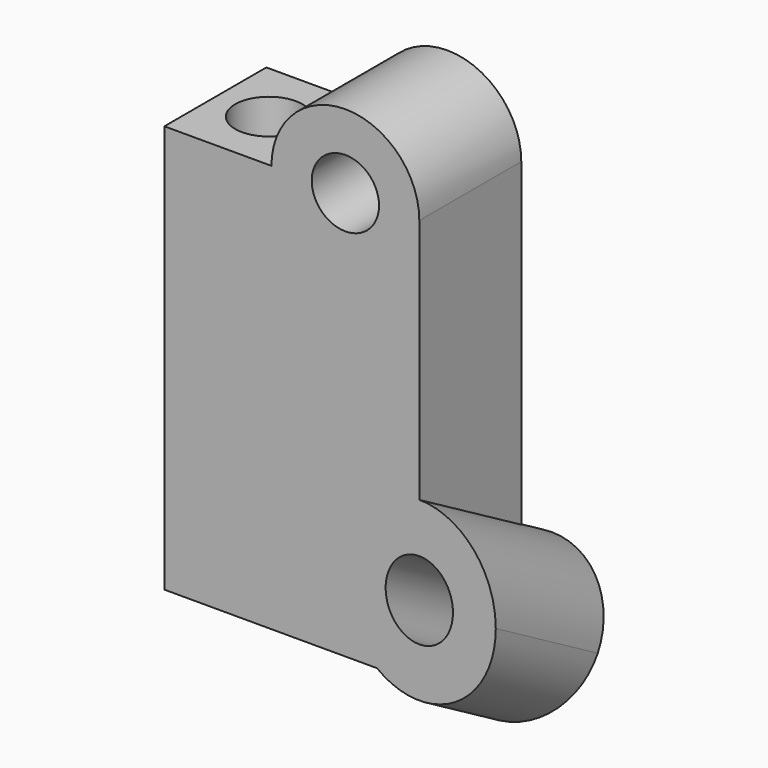
from build123d import *

# Parameters (mm, degrees)
F1_DEPTH        = 25
F3_R            = 15
F4_DEPTH        = 52
F6_D            = 13.2
F6_CBORE_D      = 19.25
F6_CBORE_DEPTH  = 0
F8_D            = 13.2
F8_CBORE_D      = 19.25
F8_CBORE_DEPTH  = 0
F10_D           = 13.2
F10_CBORE_D     = 19.25
F10_CBORE_DEPTH = 0
F11_W           = 35.8968544751
F11_H           = 52.9583077878
F12_DEPTH       = 58


with BuildPart() as f1:
    # F0 (on Front) → F1 (new body)
    with BuildSketch(Plane.XZ):
        with BuildLine():
            Line((-25, -40), (25, -40))
            Line((25, -40), (25, 40))
            ThreePointArc((25, 40), (10.5, 25.5), (-4, 40))
            Line((-4, 40), (-25, 40))
            Line((-25, 40), (-25, -40))
        make_face()
        with BuildLine():
            ThreePointArc((-4, 40), (10.5, 25.5), (25, 40))
            Line((25, 40), (-4, 40))
        make_face()
        with BuildLine():
            Line((-4, 40), (25, 40))
            ThreePointArc((25, 40), (10.5, 54.5), (-4, 40))
        make_face()
    extrude(amount=F1_DEPTH)

    # F3 (on face) → F4 (join)
    with BuildSketch(Plane(origin=(0, 17.3205080757, -10), x_dir=(1, 0, 0), z_dir=(0, -0.8660254038, 0.5))):
        with Locations((25, -34.6410161514)):
            Circle(F3_R)
    extrude(amount=F4_DEPTH)

    # F6 (through all)
    with Locations(Plane(origin=(0, 17.3205080757, -10), x_dir=(-1, 0, 0), z_dir=(0, 0.8660254038, -0.5))):
        with Locations((-25, -34.6410161514)):
            CounterBoreHole(F6_D / 2, F6_CBORE_D / 2, F6_CBORE_DEPTH)

    # F8 (through all)
    with Locations(Plane(origin=(0, 0, 0), x_dir=(-1, 0, 0), z_dir=(0, 1, 0))):
        with Locations((-10.5, 40)):
            CounterBoreHole(F8_D / 2, F8_CBORE_D / 2, F8_CBORE_DEPTH)

    # F10 (through all)
    with Locations(Plane.XY.offset(40)):
        with Locations((-14.5, -12.5)):
            CounterBoreHole(F10_D / 2, F10_CBORE_D / 2, F10_CBORE_DEPTH)

    # F11 (on Right) → F12 (cut)
    with BuildSketch(Plane.YZ):
        with Locations((-42.9484272376, -22.4903533235)):
            Rectangle(F11_W, F11_H)
    extrude(amount=F12_DEPTH, mode=Mode.SUBTRACT)


solid = f1.part
